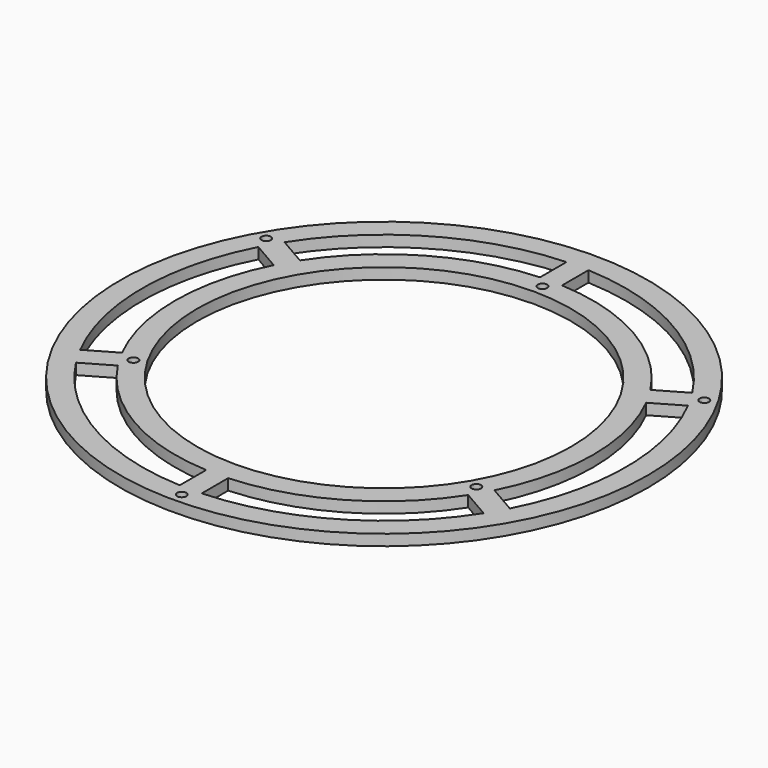
from build123d import *

# Parameters (mm, degrees)
F0_R            = 76.2
F0_R_2          = 1.35255
F0_R_3          = 53.975
F1_DEPTH        = 3.175
F3_DEPTH        = 3.175
F3_COPIES_COUNT = 6


# Not quite as in the source:
# - a pattern or mirror of a feature is missing from the dataset's text; its kind, count and spacing are read off the source's solid


with BuildPart() as f1:
    # F0 (on Top) → F1 (new body)
    with BuildSketch(Plane.XY):
        Circle(F0_R)
        with Locations((-49.4933518263, -28.575)):
            Circle(F0_R_2, mode=Mode.SUBTRACT)
        with Locations((0, -73.025)):
            Circle(F0_R_2, mode=Mode.SUBTRACT)
        with Locations((49.4933518263, -28.575)):
            Circle(F0_R_2, mode=Mode.SUBTRACT)
        with Locations((-63.2415051114, 36.5125)):
            Circle(F0_R_2, mode=Mode.SUBTRACT)
        Circle(F0_R_3, mode=Mode.SUBTRACT)
        with Locations((63.2415051114, 36.5125)):
            Circle(F0_R_2, mode=Mode.SUBTRACT)
        with Locations((0, 57.15)):
            Circle(F0_R_2, mode=Mode.SUBTRACT)
    extrude(amount=F1_DEPTH)

    # F2 (on face) → F3 (cut, through all)
    with BuildSketch(Plane.XY.offset(3.175)):
        with BuildLine():
            ThreePointArc((-53.7580736024, -27.3710640561), (-60.325, 0), (-53.7580736024, 27.3710640561))
            Line((-53.7580736024, 27.3710640561), (-62.0168505364, 32.1392711421))
            ThreePointArc((-62.0168505364, 32.1392711421), (-69.85, 0), (-62.0168505364, -32.1392711421))
            Line((-62.0168505364, -32.1392711421), (-53.7580736024, -27.3710640561))
        make_face()
    f3 = extrude(amount=-F3_DEPTH, mode=Mode.SUBTRACT)

    # F3_copies: F3 ×6 about axis
    f3_copies_axis = Axis((0, 0, 0), (0, 0, 1))
    for i in range(1, F3_COPIES_COUNT):
        add(f3.rotate(f3_copies_axis, i * 360 / F3_COPIES_COUNT), mode=Mode.SUBTRACT)


solid = f1.part
